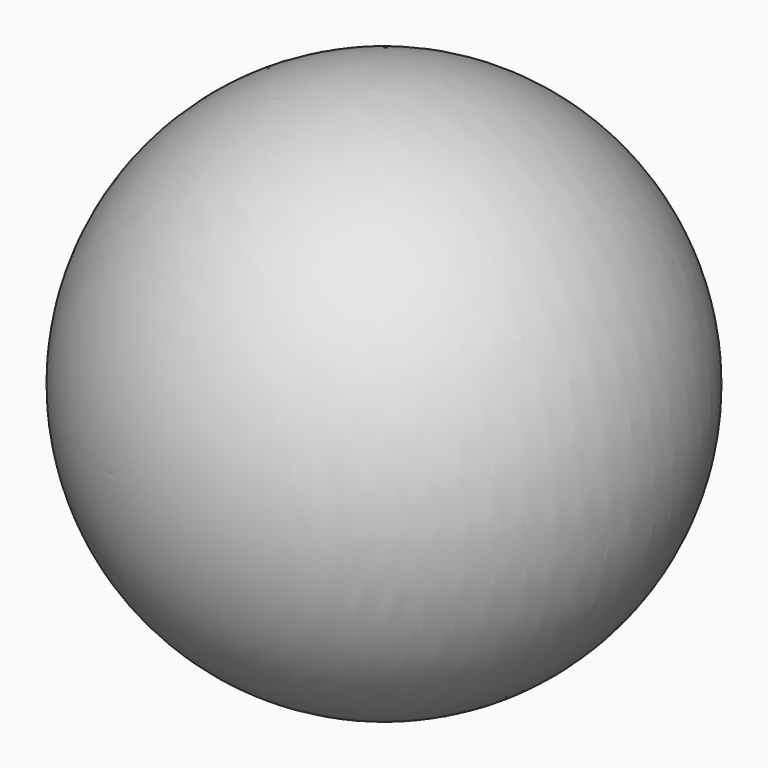
from build123d import *


with BuildPart() as f2:
    # F1 (on face) → F2 (revolve)
    with BuildSketch(Plane.XY):
        with BuildLine():
            ThreePointArc((-34.8645252768, 82.5636375234), (-100.295698042, 40.5005522972), (-57.9646417795, -24.7575750424))
            Line((-57.9646417795, -24.7575750424), (-34.8645252768, 82.5636375234))
        make_face()
    revolve(axis=Axis((-46.33737728, 29.2617250234, 0), (0.2104235647, 0.9776103127, 0)))


solid = f2.part
